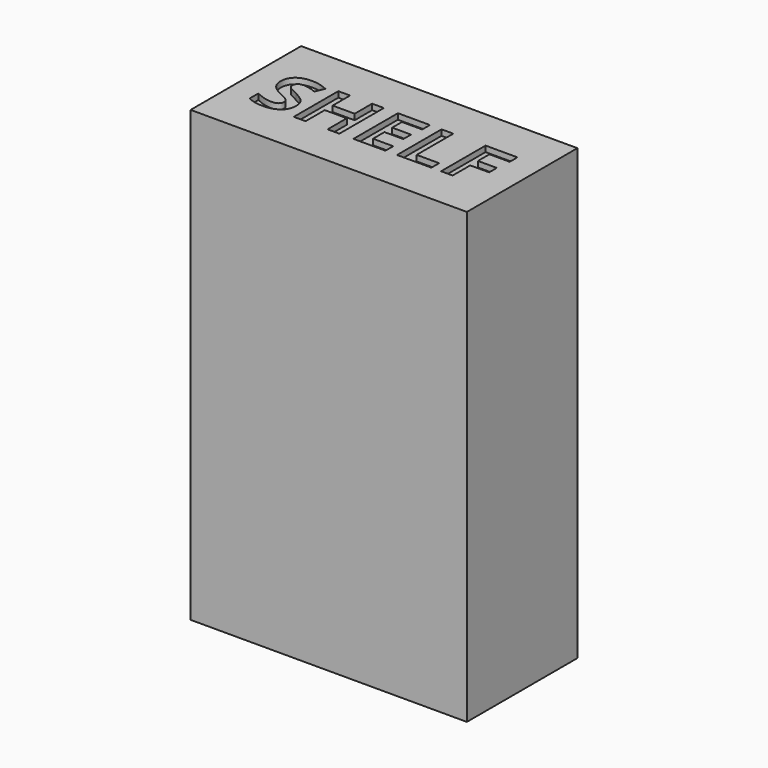
from build123d import *

# Parameters (mm, degrees)
F0_W         = 1219.2
F0_H         = 609.6
F1_DEPTH     = 1981.2
F2_TEXT_SIZE = 343.8282551037
F3_DEPTH     = 25.4


# Not quite as in the source:
# - Text() gives the source's letters only with a copy of the font that has no kerning and outlines rounded to 1/6400 em; it was checked with that copy


with BuildPart() as f1:
    # F0 (on Top) → F1 (new body)
    with BuildSketch(Plane.XY):
        with Locations((609.6, 304.8)):
            Rectangle(F0_W, F0_H)
    extrude(amount=F1_DEPTH)

    # F2 (on face) → F3 (cut)
    with BuildSketch(Plane.XY.offset(1981.2)):
        with Locations((89.8872315884, 181.4527958632)):
            Text('SHELF', F2_TEXT_SIZE, font='Open Sans', font_style=FontStyle.BOLD, text_align=(TextAlign.LEFT, TextAlign.BOTTOM))
    extrude(amount=-F3_DEPTH, mode=Mode.SUBTRACT)


solid = f1.part
